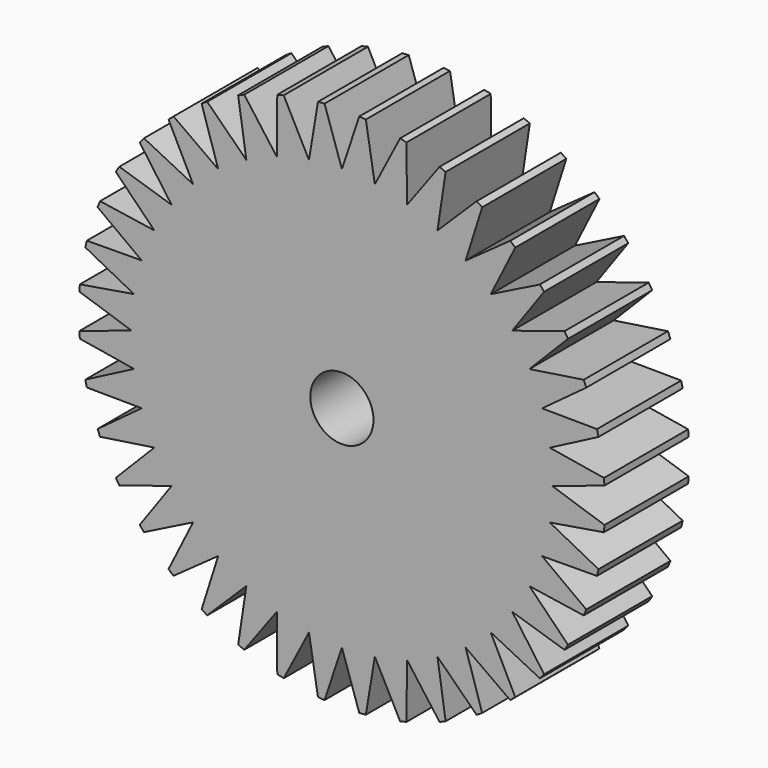
from build123d import *

# Parameters (mm, degrees)
F0_R            = 25
F0_R_2          = 3
F1_DEPTH        = 10
F3_DEPTH        = 25
F3_COPIES_COUNT = 40


# Not quite as in the source:
# - a pattern or mirror of a feature is missing from the dataset's text; its kind, count and spacing are read off the source's solid


with BuildPart() as f1:
    # F0 (on Front) → F1 (new body)
    with BuildSketch(Plane.XZ):
        Circle(F0_R)
        Circle(F0_R_2, mode=Mode.SUBTRACT)
    extrude(amount=F1_DEPTH)

    # F2 (on face) → F3 (cut)
    with BuildSketch(Plane.XZ.offset(10)):
        Polygon((2, 26), (-2, 26), (0, 20), align=None)
    f3 = extrude(amount=-F3_DEPTH, mode=Mode.SUBTRACT)

    # F3_copies: F3 ×40 about axis
    f3_copies_axis = Axis((0, 0, 0), (0, 1, 0))
    for i in range(1, F3_COPIES_COUNT):
        add(f3.rotate(f3_copies_axis, i * 360 / F3_COPIES_COUNT), mode=Mode.SUBTRACT)


solid = f1.part
